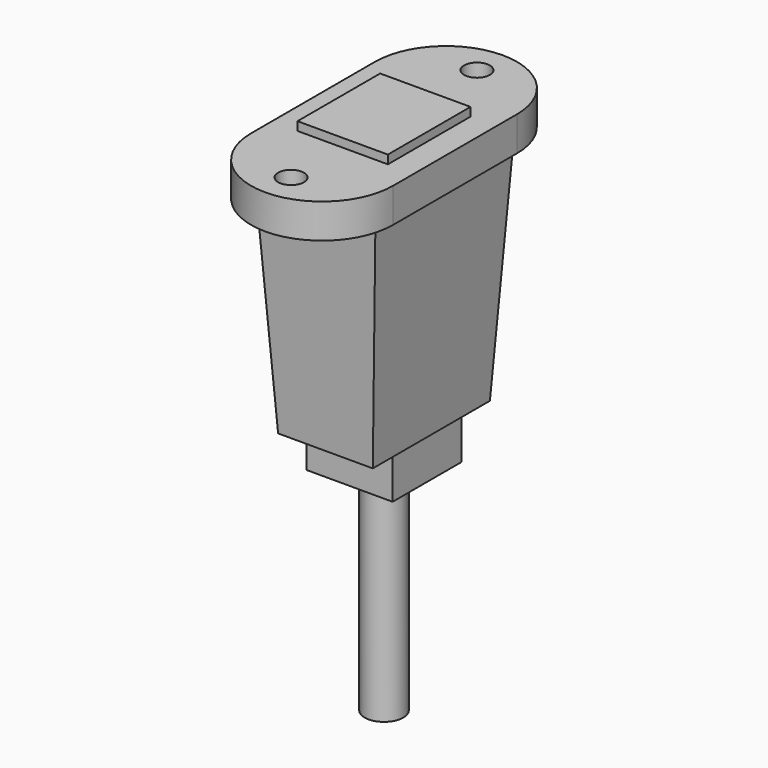
from build123d import *

# Parameters (mm, degrees)
F0_W      = 16.5
F0_H      = 18
F0_W_2    = 10.5
F0_H_2    = 12
F0_R      = 1.5
F1_DEPTH  = 4
F2_W      = 14
F2_H      = 20
F3_DEPTH  = 26
F4_SIZE2  = 25.99999
F4_SIZE   = 1.49999
F5_W      = 10
F5_H      = 10
F6_DEPTH  = 5
F7_R      = 2.25
F8_DEPTH  = 25
F9_W      = 10.5
F9_H      = 12
F10_DEPTH = 1


# Not quite as in the source:
# - a fillet or chamfer is up to 0.001 mm smaller than in the source, because OpenCascade refuses the exact size


with BuildPart() as f1:
    # F0 (on Top) → F1 (new body)
    with BuildSketch(Plane.XY):
        Rectangle(F0_W, F0_H)
        Rectangle(F0_W_2, F0_H_2, mode=Mode.SUBTRACT)
        with BuildLine():
            Line((-8.25, 9), (8.25, 9))
            ThreePointArc((8.25, 9), (0, 17.25), (-8.25, 9))
        make_face()
        with Locations((0, 13.5)):
            Circle(F0_R, mode=Mode.SUBTRACT)
        with BuildLine():
            ThreePointArc((-8.25, -9), (0, -17.25), (8.25, -9))
            Line((8.25, -9), (-8.25, -9))
        make_face()
        with Locations((0, -13.5)):
            Circle(F0_R, mode=Mode.SUBTRACT)
    extrude(amount=-F1_DEPTH)

    # F2 (on face) → F3 (join)
    with BuildSketch(Plane(origin=(0, 0, -4), x_dir=(1, 0, 0), z_dir=(0, 0, -1))):
        Rectangle(F2_W, F2_H)
    extrude(amount=F3_DEPTH)

    # F4 (size 1.5 and 26 in the source; OpenCascade refuses exactly that, so slightly less here)
    f4_edges = [f1.edges().sort_by_distance(p)[0] for p in [
        (0, -10, -30),
        (0, 10, -30),
        (7, 0, -30),
        (-7, 0, -30),
    ]]
    f4_side = f1.faces().sort_by_distance((0, 0, -30))[0]
    chamfer(f4_edges, length=F4_SIZE, length2=F4_SIZE2, reference=f4_side)

    # F5 (on face) → F6 (join)
    with BuildSketch(Plane(origin=(0, 0, -30), x_dir=(1, 0, 0), z_dir=(0, 0, -1))):
        Rectangle(F5_W, F5_H)
    extrude(amount=F6_DEPTH)

    # F7 (on face) → F8 (join)
    with BuildSketch(Plane(origin=(0, 0, -35), x_dir=(1, 0, 0), z_dir=(0, 0, -1))):
        Circle(F7_R)
    extrude(amount=F8_DEPTH)

    # F9 (on face) → F10 (join)
    with BuildSketch(Plane.XY):
        Rectangle(F9_W, F9_H)
    extrude(amount=F10_DEPTH)


solid = f1.part
